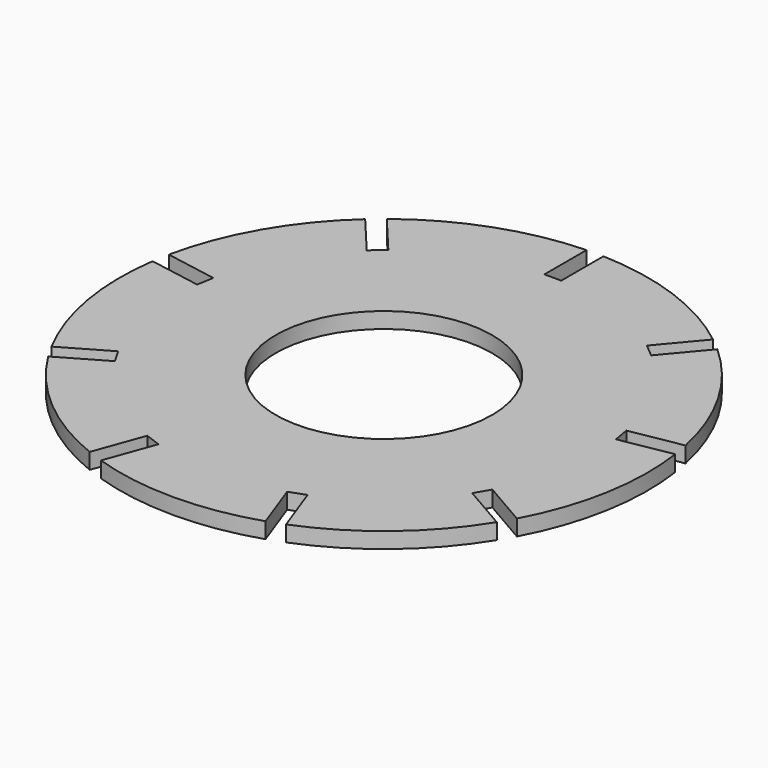
from build123d import *

# Parameters (mm, degrees)
F0_R            = 50
F0_R_2          = 20.5
F1_DEPTH        = 3
F2_W            = 3.2
F2_H            = 40
F3_DEPTH        = 25
F3_COPIES_COUNT = 9


# Not quite as in the source:
# - a pattern or mirror of a feature is missing from the dataset's text; its kind, count and spacing are read off the source's solid


with BuildPart() as f1:
    # F0 (on Top) → F1 (new body)
    with BuildSketch(Plane.XY):
        Circle(F0_R)
        Circle(F0_R_2, mode=Mode.SUBTRACT)
    extrude(amount=F1_DEPTH)

    # F2 (on face) → F3 (cut)
    with BuildSketch(Plane.XY.offset(3)):
        with Locations((0, 60)):
            Rectangle(F2_W, F2_H)
    f3 = extrude(amount=-F3_DEPTH, mode=Mode.SUBTRACT)

    # F3_copies: F3 ×9 about axis
    f3_copies_axis = Axis((0, 0, 0), (0, 0, 1))
    for i in range(1, F3_COPIES_COUNT):
        add(f3.rotate(f3_copies_axis, i * 360 / F3_COPIES_COUNT), mode=Mode.SUBTRACT)


solid = f1.part
